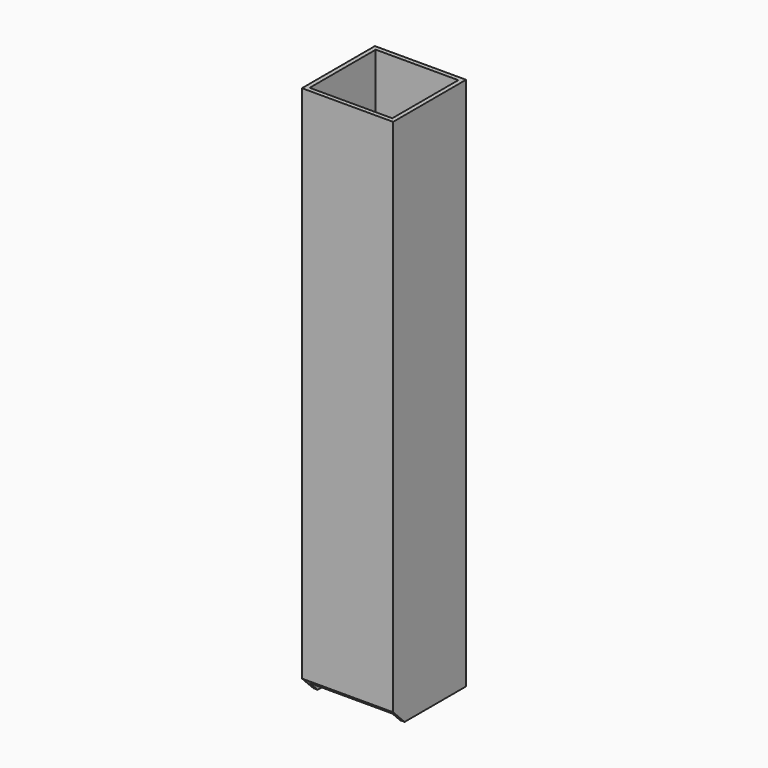
from build123d import *

# Parameters (mm, degrees)
F0_W        = 63.5
F0_H        = 63.5
F0_W_2      = 57.5
F0_H_2      = 57.5
F1_DEPTH    = 372
F2_T1_DEPTH = 114.9336597593


# Not quite as in the source:
# - a fillet or chamfer that OpenCascade refuses, or shapes differently, is made with other operations: its cross-section is extruded or revolved along the edge and cut away or added


with BuildPart() as f1:
    # F0 (on Top) → F1 (new body)
    with BuildSketch(Plane.XY):
        with Locations((4.6706348658, 6.1677011834)):
            Rectangle(F0_W, F0_H)
        with Locations((4.6706348658, 6.1677011834)):
            Rectangle(F0_W_2, F0_H_2, mode=Mode.SUBTRACT)
    extrude(amount=F1_DEPTH)

    # F2: chamfer of 10 on 1 edges, made by hand

    # F2_s2 → F2_t1 (cut)
    with BuildSketch(Plane.YZ.offset(-52.7961950139)):
        Polygon((-25.5822988166, 10), (-15.5822988166, 0), (-25.5822988166, 0), align=None)
    extrude(amount=F2_T1_DEPTH, mode=Mode.SUBTRACT)


solid = f1.part
